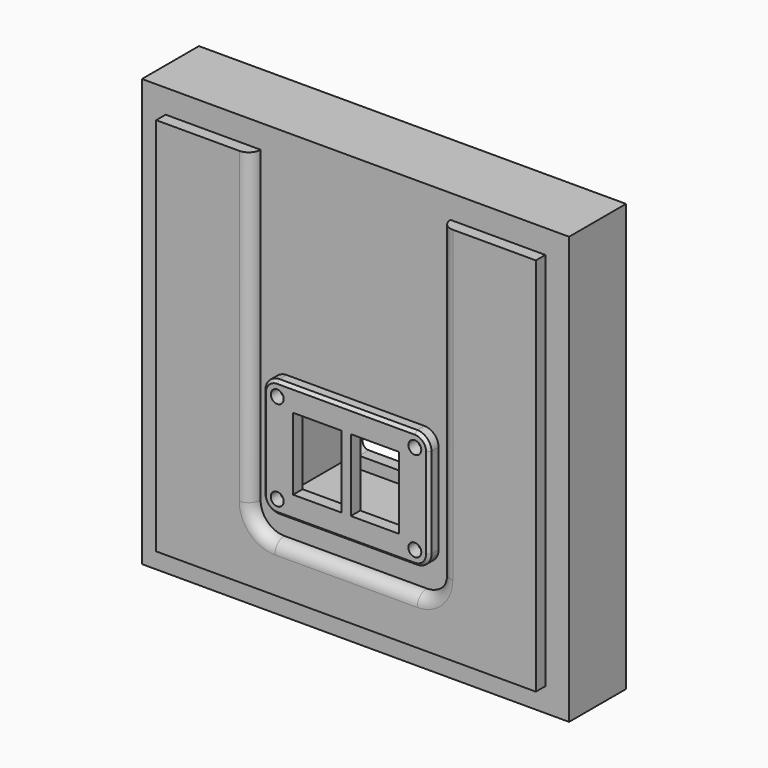
from build123d import *

# Parameters (mm, degrees)
F0_W      = 114.3
F0_H      = 114.3
F1_DEPTH  = 19.05
F3_DEPTH  = 3.175
F4_R      = 3.17499
F5_W      = 38.1
F5_H      = 25.4
F6_DEPTH  = 19.051
F8_DEPTH  = 3.175
F9_SIZE   = 0.79375
F10_W     = 12.9032
F10_H     = 19.304
F11_DEPTH = 22.226
F12_R     = 1.7272
F13_DEPTH = 22.226
F14_R     = 1.7272
F15_DEPTH = 3.175


# Not quite as in the source:
# - a fillet or chamfer is up to 0.001 mm smaller than in the source, because OpenCascade refuses the exact size


with BuildPart() as f1:
    # F0 (on Front) → F1 (new body)
    with BuildSketch(Plane.XZ):
        Rectangle(F0_W, F0_H)
    extrude(amount=-F1_DEPTH)

    # F5 (on Front) → F6 (cut, through all)
    with BuildSketch(Plane.XZ):
        with Locations((0, -15.875)):
            Rectangle(F5_W, F5_H)
    extrude(amount=-F6_DEPTH, mode=Mode.SUBTRACT)


with BuildPart() as f3:
    # F2 (on Front) → F3 (new body)
    with BuildSketch(Plane.XZ):
        with BuildLine():
            Line((-50.8, 50.8), (-50.8, -50.8))
            Line((-50.8, -50.8), (50.8, -50.8))
            Line((50.8, -50.8), (50.8, 50.8))
            Line((50.8, 50.8), (25.4, 50.8))
            Line((25.4, 50.8), (25.4, -31.75))
            ThreePointArc((25.4, -31.75), (23.5401280605, -36.2401280605), (19.05, -38.1))
            Line((19.05, -38.1), (-19.05, -38.1))
            ThreePointArc((-19.05, -38.1), (-23.5401280605, -36.2401280605), (-25.4, -31.75))
            Line((-25.4, -31.75), (-25.4, 50.8))
            Line((-25.4, 50.8), (-50.8, 50.8))
        make_face()
    extrude(amount=F3_DEPTH)

    # F4 (radius 3.175 in the source; OpenCascade refuses exactly that, so slightly less here)
    f4_edges = [f3.edges().sort_by_distance(p)[0] for p in [
        (-25.4, -3.175, 9.525),
        (25.4, -3.175, 9.525),
        (23.540128, -3.175, -36.240128),
        (0, -3.175, -38.1),
        (-23.540128, -3.175, -36.240128),
    ]]
    fillet(f4_edges, radius=F4_R)


with BuildPart() as f8:
    # F7 (on Front) → F8 (new body)
    with BuildSketch(Plane.XZ):
        with BuildLine():
            Line((18.40865, 0), (-18.40865, 0))
            ThreePointArc((-18.40865, 0), (-21.1072169644, -1.1177830356), (-22.225, -3.81635))
            Line((-22.225, -3.81635), (-22.225, -27.93365))
            ThreePointArc((-22.225, -27.93365), (-21.1072169644, -30.6322169644), (-18.40865, -31.75))
            Line((-18.40865, -31.75), (18.40865, -31.75))
            ThreePointArc((18.40865, -31.75), (21.1072169644, -30.6322169644), (22.225, -27.93365))
            Line((22.225, -27.93365), (22.225, -3.81635))
            ThreePointArc((22.225, -3.81635), (21.1072169644, -1.1177830356), (18.40865, 0))
        make_face()
    extrude(amount=F8_DEPTH)

    # F9
    f9_edges = [f8.edges().sort_by_distance(p)[0] for p in [
        (0, -3.175, 0),
        (-21.107217, -3.175, -1.117783),
        (-22.225, -3.175, -15.875),
        (-21.107217, -3.175, -30.632217),
        (0, -3.175, -31.75),
        (21.107217, -3.175, -30.632217),
        (22.225, -3.175, -15.875),
        (21.107217, -3.175, -1.117783),
    ]]
    chamfer(f9_edges, length=F9_SIZE)

    # F10 (on face) → F11 (cut, through all)
    with BuildSketch(Plane.XZ.offset(3.175)):
        with Locations((-7.7216, -15.875)):
            Rectangle(F10_W, F10_H)
        with Locations((7.7216, -15.875)):
            Rectangle(F10_W, F10_H)
    extrude(amount=-F11_DEPTH, mode=Mode.SUBTRACT)

    # F12 (on face) → F13 (cut, through all)
    with BuildSketch(Plane.XZ.offset(3.175)):
        with Locations((-18.40865, -3.81635)):
            Circle(F12_R)
        with Locations((-18.40865, -27.93365)):
            Circle(F12_R)
        with Locations((18.40865, -3.81635)):
            Circle(F12_R)
        with Locations((18.40865, -27.93365)):
            Circle(F12_R)
    extrude(amount=-F13_DEPTH, mode=Mode.SUBTRACT)


with BuildPart() as f15:
    # F14 (on face) → F15 (new body)
    with BuildSketch(Plane(origin=(0, 19.05, 0), x_dir=(-1, 0, 0), z_dir=(0, 1, 0))):
        with BuildLine():
            Line((22.2250037253, 3.175), (-22.2249962747, 3.175))
            ThreePointArc((-22.2249962747, 3.175), (-24.470060305, 2.2450640303), (-25.3999962747, 0))
            Line((-25.3999962747, 0), (-25.3999962747, -31.75))
            ThreePointArc((-25.3999962747, -31.75), (-24.470060305, -33.9950640303), (-22.2249962747, -34.925))
            Line((-22.2249962747, -34.925), (22.2250037253, -34.925))
            ThreePointArc((22.2250037253, -34.925), (24.4700677556, -33.9950640303), (25.4000037253, -31.75))
            Line((25.4000037253, -31.75), (25.4000037253, 0))
            ThreePointArc((25.4000037253, 0), (24.4700677556, 2.2450640303), (22.2250037253, 3.175))
        make_face()
        with Locations((-18.40865, -27.93365)):
            Circle(F14_R, mode=Mode.SUBTRACT)
        with Locations((18.40865, -27.93365)):
            Circle(F14_R, mode=Mode.SUBTRACT)
        with BuildLine():
            ThreePointArc((-15.875, -7.9375), (-15.4100320151, -6.8149679849), (-14.2875, -6.35))
            Line((-14.2875, -6.35), (14.2875, -6.35))
            ThreePointArc((14.2875, -6.35), (15.4100320151, -6.8149679849), (15.875, -7.9375))
            Line((15.875, -7.9375), (15.875, -23.8125))
            ThreePointArc((15.875, -23.8125), (15.4100320151, -24.9350320151), (14.2875, -25.4))
            Line((14.2875, -25.4), (-14.2875, -25.4))
            ThreePointArc((-14.2875, -25.4), (-15.4100320151, -24.9350320151), (-15.875, -23.8125))
            Line((-15.875, -23.8125), (-15.875, -7.9375))
        make_face(mode=Mode.SUBTRACT)
        with Locations((-18.40865, -3.81635)):
            Circle(F14_R, mode=Mode.SUBTRACT)
        with Locations((18.40865, -3.81635)):
            Circle(F14_R, mode=Mode.SUBTRACT)
    extrude(amount=F15_DEPTH)


solid = Compound([f1.part, f3.part, f8.part, f15.part])
